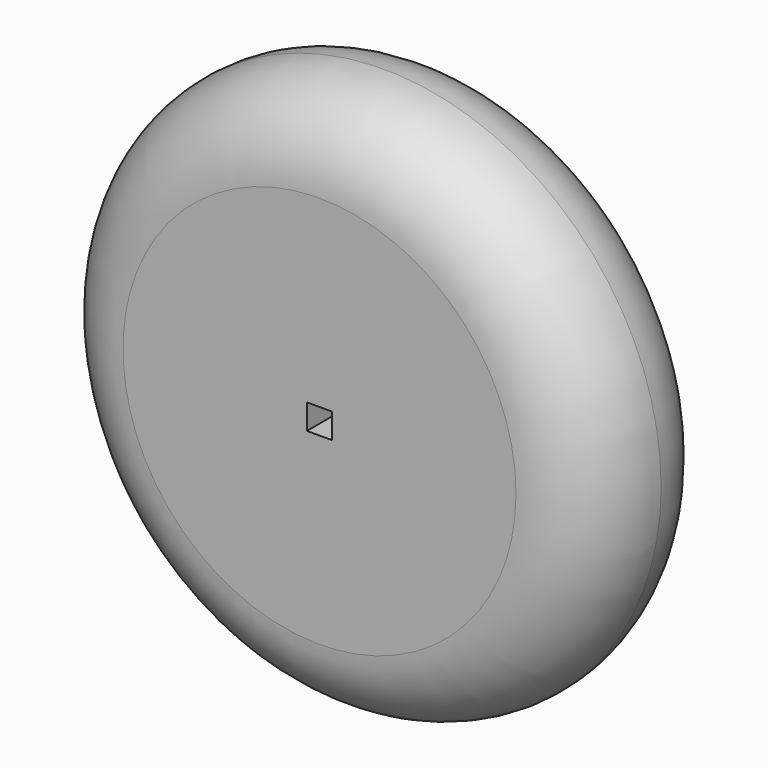
from build123d import *

# Parameters (mm, degrees)
F0_R     = 34.925
F1_DEPTH = 20.32
F2_R     = 10.15999
F3_W     = 3.175
F3_H     = 3.175
F4_DEPTH = 20.32


# Not quite as in the source:
# - a fillet or chamfer is up to 0.001 mm smaller than in the source, because OpenCascade refuses the exact size


with BuildPart() as f1:
    # F0 (on Front) → F1 (new body)
    with BuildSketch(Plane.XZ):
        Circle(F0_R)
    extrude(amount=F1_DEPTH)

    # F2 (radius 10.16 in the source; OpenCascade refuses exactly that, so slightly less here)
    f2_edges = [f1.edges().sort_by_distance(p)[0] for p in [
        (-34.925, -20.32, 0),
        (-34.925, 0, 0),
    ]]
    fillet(f2_edges, radius=F2_R)

    # F3 (on face) → F4 (cut, through all)
    with BuildSketch(Plane.XZ.offset(20.32)):
        Rectangle(F3_W, F3_H)
    extrude(amount=-F4_DEPTH, mode=Mode.SUBTRACT)


solid = f1.part
